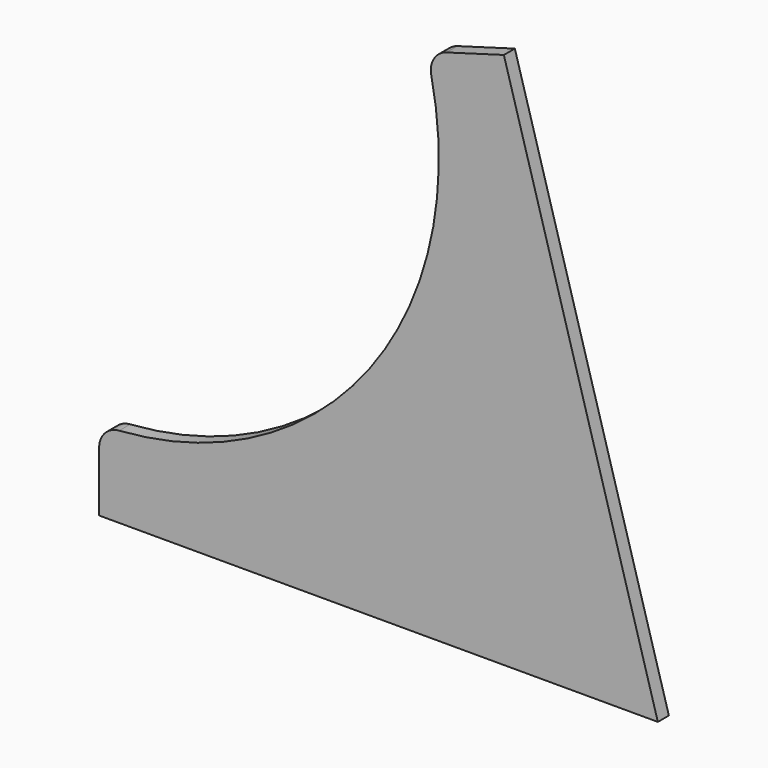
from build123d import *

# Parameters (mm, degrees)
F1_DEPTH = 1.6
F2_R     = 2.5


with BuildPart() as f1:
    # F0 (on Front) → F1 (new body)
    with BuildSketch(Plane.XZ):
        with BuildLine():
            Line((-65, 0), (0, 0))
            Line((0, 0), (-17.9164281281, 62.482010236))
            Line((-17.9164281281, 62.482010236), (-26.9059650358, 59.9043020076))
            ThreePointArc((-26.9059650358, 59.9043020076), (-33.542691422, 25.2762309724), (-65, 9.3518101738))
            Line((-65, 9.3518101738), (-65, 0))
        make_face()
    extrude(amount=F1_DEPTH)

    # F2
    f2_edges = [f1.edges().sort_by_distance(p)[0] for p in [
        (-26.905965, -0.8, 59.904302),
        (-65, -0.8, 9.35181),
    ]]
    fillet(f2_edges, radius=F2_R)


solid = f1.part
